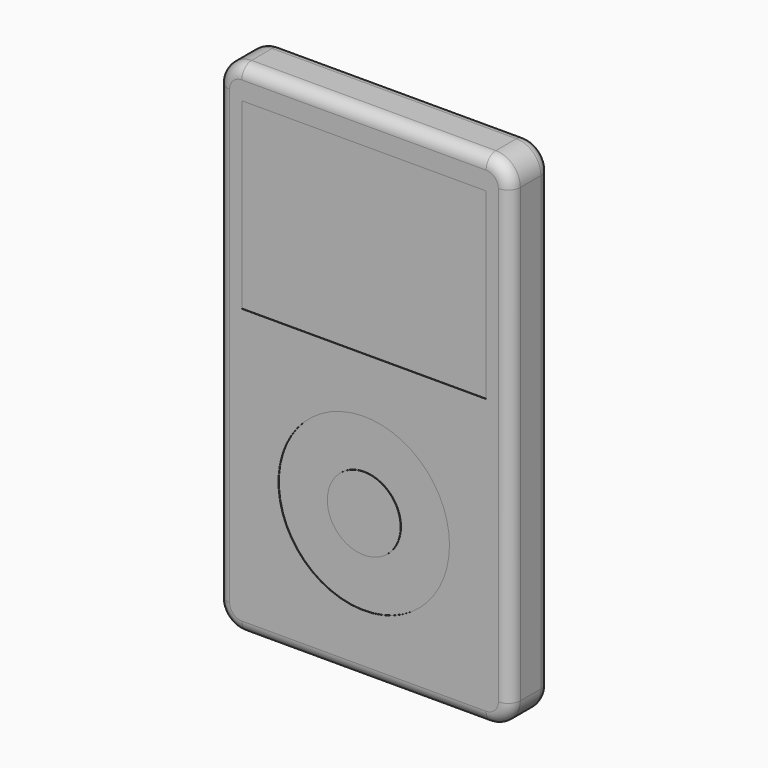
from build123d import *

# Parameters (mm, degrees)
F0_R     = 17.78
F0_W     = 50.8
F0_H     = 38.1
F0_R_2   = 7.62
F1_DEPTH = 10.414
F2_DEPTH = 0.1
F3_W     = 10.16
F3_H     = 2.54
F3_R     = 2.54
F3_W_2   = 20.32
F4_DEPTH = 1
F5_R     = 2.54


with BuildPart() as f1:
    # F0 (on Front) → F1 (new body)
    with BuildSketch(Plane.XZ):
        with BuildLine():
            ThreePointArc((30.48, 46.99), (28.9921024484, 50.5821024484), (25.4, 52.07))
            Line((25.4, 52.07), (-25.4, 52.07))
            ThreePointArc((-25.4, 52.07), (-28.9921024484, 50.5821024484), (-30.48, 46.99))
            Line((-30.48, 46.99), (-30.48, -46.99))
            ThreePointArc((-30.48, -46.99), (-28.9921024484, -50.5821024484), (-25.4, -52.07))
            Line((-25.4, -52.07), (25.4, -52.07))
            ThreePointArc((25.4, -52.07), (28.9921024484, -50.5821024484), (30.48, -46.99))
            Line((30.48, -46.99), (30.48, 46.99))
        make_face()
        with Locations((0, -21.59)):
            Circle(F0_R, mode=Mode.SUBTRACT)
        with Locations((0, 26.67)):
            Rectangle(F0_W, F0_H, mode=Mode.SUBTRACT)
        with Locations((0, 26.67)):
            Rectangle(F0_W, F0_H)
        with Locations((0, -21.59)):
            Circle(F0_R)
        with Locations((0, -21.59)):
            Circle(F0_R_2, mode=Mode.SUBTRACT)
        with Locations((0, -21.59)):
            Circle(F0_R_2)
    extrude(amount=-F1_DEPTH)

    # F0 (on Front) → F2 (cut)
    with BuildSketch(Plane.XZ):
        with Locations((0, 26.67)):
            Rectangle(F0_W, F0_H)
        with Locations((0, -21.59)):
            Circle(F0_R)
        with Locations((0, -21.59)):
            Circle(F0_R_2, mode=Mode.SUBTRACT)
    extrude(amount=-F2_DEPTH, mode=Mode.SUBTRACT)

    # F3 (on face) → F4 (cut)
    with BuildSketch(Plane(origin=(0, 10.414, 0), x_dir=(-1, 0, 0), z_dir=(0, 1, 0))):
        with Locations((-20.32, 44.45)):
            Rectangle(F3_W, F3_H)
        with Locations((21.59, 43.18)):
            Circle(F3_R)
        with Locations((0, -45.72)):
            Rectangle(F3_W_2, F3_H)
    extrude(amount=-F4_DEPTH, mode=Mode.SUBTRACT)

    # F5
    f5_edges = [f1.edges().sort_by_distance(p)[0] for p in [
        (30.48, 0, 0),
        (30.48, 10.414, 0),
    ]]
    fillet(f5_edges, radius=F5_R)


solid = f1.part
